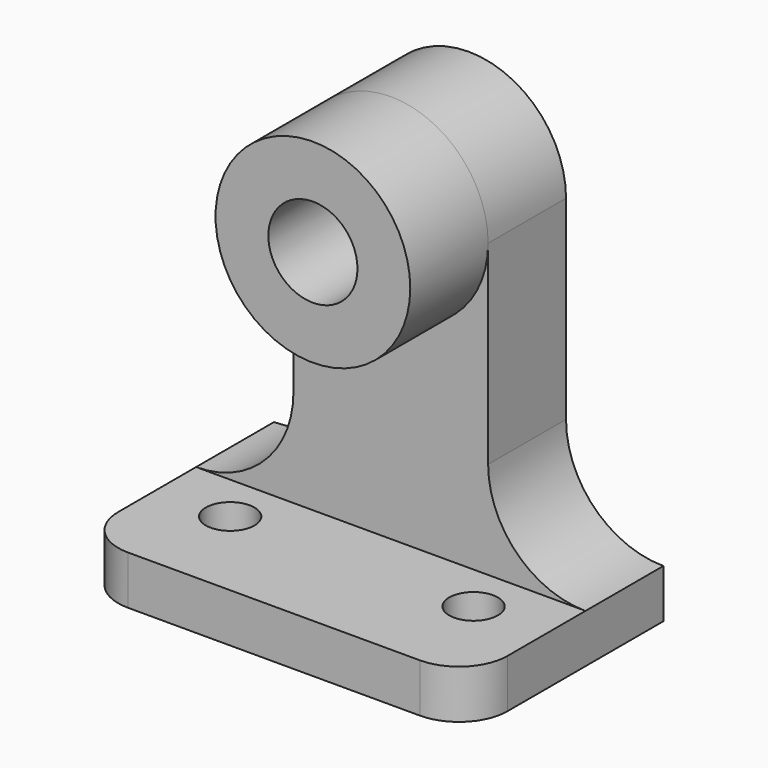
from build123d import *

# Parameters (mm, degrees)
F0_W      = 50.8
F0_H      = 31.75
F1_DEPTH  = 6.35
F3_DEPTH  = 25.4
F4_W      = 50.8
F4_H      = 12.7
F5_DEPTH  = 38.1
F6_R      = 3.175
F7_DEPTH  = 25.4
F9_DEPTH  = 25.4
F10_DEPTH = 25.4
F12_DEPTH = 12.7
F14_DEPTH = 12.7
F15_R     = 5.8141785566
F16_DEPTH = 19.05


# Not quite as in the source:
# - a feature names something its author has since deleted; it is built from what else it names


with BuildPart() as f1:
    # F0 (on Top) → F1 (new body)
    with BuildSketch(Plane.XY):
        with Locations((25.4, 15.875)):
            Rectangle(F0_W, F0_H)
    extrude(amount=F1_DEPTH)

    # F2 (on face) → F3 (cut)
    with BuildSketch(Plane.XY.offset(6.35)):
        with BuildLine():
            ThreePointArc((6.35, 0), (1.8598719395, 1.8598719395), (0, 6.35))
            Line((0, 6.35), (0, 0))
            Line((0, 0), (6.35, 0))
        make_face()
        with BuildLine():
            ThreePointArc((50.8, 6.35), (48.9401280605, 1.8598719395), (44.45, 0))
            Line((44.45, 0), (50.8, 0))
            Line((50.8, 0), (50.8, 6.35))
        make_face()
    extrude(amount=-F3_DEPTH, mode=Mode.SUBTRACT)

    # F4 (on face) → F5 (join)
    with BuildSketch(Plane.XY.offset(6.35)):
        with Locations((25.4, 25.4)):
            Rectangle(F4_W, F4_H)
    extrude(amount=F5_DEPTH)

    # F6 (on face) → F7 (cut)
    with BuildSketch(Plane.XY.offset(6.35)):
        with Locations((9.525, 12.7)):
            Circle(F6_R)
        with Locations((41.275, 12.7)):
            Circle(F6_R)
    extrude(amount=-F7_DEPTH, mode=Mode.SUBTRACT)

    # F8 (on face) → F9 (cut)
    with BuildSketch(Plane.XZ.offset(-19.05)):
        with BuildLine():
            Line((12.7, 19.05), (12.7, 44.45))
            Line((12.7, 44.45), (0, 44.45))
            Line((0, 44.45), (0, 6.35))
            ThreePointArc((0, 6.35), (8.9802561211, 10.0697438789), (12.7, 19.05))
        make_face()
        with BuildLine():
            Line((50.8, 44.45), (38.1, 44.45))
            Line((38.1, 44.45), (38.1, 19.05))
            ThreePointArc((38.1, 19.05), (41.8197438789, 10.0697438789), (50.8, 6.35))
            Line((50.8, 6.35), (50.8, 44.45))
        make_face()
    extrude(amount=-F9_DEPTH, mode=Mode.SUBTRACT)

    # F8 (on face) → F10 (cut)
    with BuildSketch(Plane.XZ.offset(-19.05)):
        with BuildLine():
            Line((12.7, 19.05), (12.7, 44.45))
            Line((12.7, 44.45), (0, 44.45))
            Line((0, 44.45), (0, 6.35))
            ThreePointArc((0, 6.35), (8.9802561211, 10.0697438789), (12.7, 19.05))
        make_face()
        with BuildLine():
            Line((38.1, 44.45), (12.7, 44.45))
            ThreePointArc((12.7, 44.45), (25.4, 31.75), (38.1, 44.45))
        make_face()
        with BuildLine():
            Line((50.8, 44.45), (38.1, 44.45))
            Line((38.1, 44.45), (38.1, 19.05))
            ThreePointArc((38.1, 19.05), (41.8197438789, 10.0697438789), (50.8, 6.35))
            Line((50.8, 6.35), (50.8, 44.45))
        make_face()
    extrude(amount=-F10_DEPTH, mode=Mode.SUBTRACT)

    # F11 (on face) → F12 (join)
    with BuildSketch(Plane.XZ.offset(-19.05)):
        with BuildLine():
            ThreePointArc((12.7, 44.45), (25.4, 31.75), (38.1, 44.45))
            ThreePointArc((38.1, 44.45), (25.4, 57.15), (12.7, 44.45))
        make_face()
    extrude(amount=-F12_DEPTH)

    # F13 (on face) → F14 (join)
    with BuildSketch(Plane.XZ.offset(-19.05)):
        with BuildLine():
            ThreePointArc((12.7, 44.45), (25.4, 31.75), (38.1, 44.45))
            ThreePointArc((38.1, 44.45), (25.4, 57.15), (12.7, 44.45))
        make_face()
    extrude(amount=F14_DEPTH)

    # F15 (on face) → F16 (cut)
    with BuildSketch(Plane.XZ.offset(-6.35)):
        with Locations((25.4, 44.45)):
            Circle(F15_R)
    extrude(amount=-F16_DEPTH, mode=Mode.SUBTRACT)


solid = f1.part
